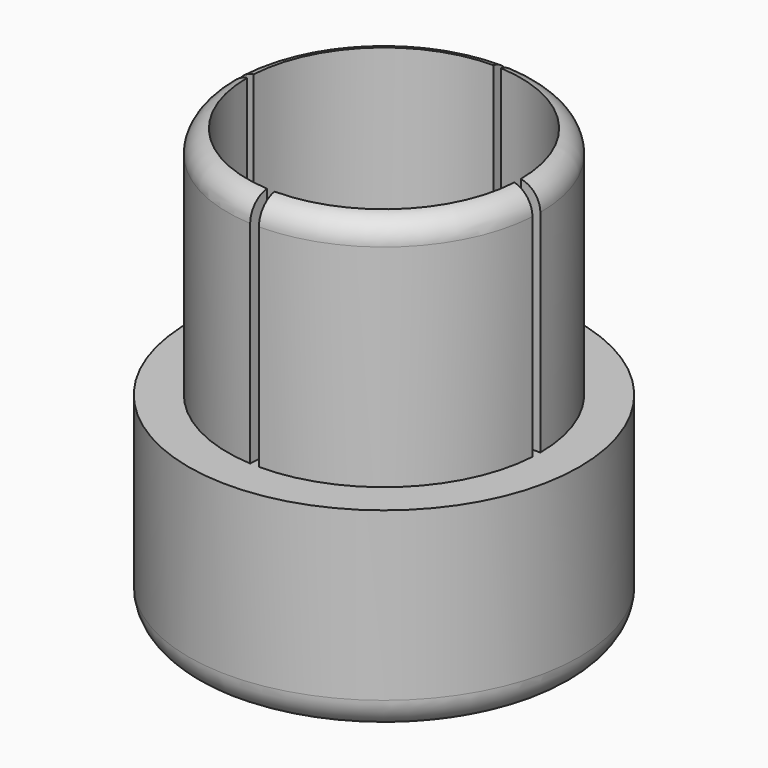
from build123d import *

# Parameters (mm, degrees)
F0_R        = 25
F0_R_2      = 20
F0_R_3      = 17.5
F1_DEPTH    = 25.4
F2_DEPTH    = 55.4
F4_DEPTH    = 30
F5_T2_ANGLE = 128.886649626
F5_T4_ANGLE = 129.1121145727
F5_T6_ANGLE = 128.886649626
F5_T8_ANGLE = 129.1121145727
F6_R        = 4


# Not quite as in the source:
# - a fillet or chamfer that OpenCascade refuses, or shapes differently, is made with other operations: its cross-section is extruded or revolved along the edge and cut away or added


with BuildPart() as f1:
    # F0 (on Top) → F1 (new body)
    with BuildSketch(Plane.XY):
        Circle(F0_R)
        Circle(F0_R_2, mode=Mode.SUBTRACT)
        Circle(F0_R_2)
        Circle(F0_R_3, mode=Mode.SUBTRACT)
    extrude(amount=F1_DEPTH)

    # F0 (on Top) → F2 (join)
    with BuildSketch(Plane.XY):
        Circle(F0_R_2)
        Circle(F0_R_3, mode=Mode.SUBTRACT)
    extrude(amount=F2_DEPTH)

    # F3 (on face) → F4 (cut)
    with BuildSketch(Plane.XY.offset(55.4)):
        with BuildLine():
            Line((0, 20), (0, 17.5))
            ThreePointArc((0, 17.5), (0.5, 17.4928556845), (0.9995917534, 17.4714285714))
            Line((0.9995917534, 17.4714285714), (1.1423905753, 19.9673469388))
            ThreePointArc((1.1423905753, 19.9673469388), (0.5714285714, 19.991835068), (0, 20))
        make_face()
        with BuildLine():
            Line((20, 0), (17.5, 0))
            ThreePointArc((17.5, 0), (17.4928556845, -0.5), (17.4714285714, -0.9995917534))
            Line((17.4714285714, -0.9995917534), (19.9626986738, -1.2209265568))
            ThreePointArc((19.9626986738, -1.2209265568), (19.9906724934, -0.6107481163), (20, 0))
        make_face()
        with BuildLine():
            ThreePointArc((-17.5, 0), (-17.4928556845, 0.5), (-17.4714285714, 0.9995917534))
            Line((-17.4714285714, 0.9995917534), (-19.9626986738, 1.2209265568))
            ThreePointArc((-19.9626986738, 1.2209265568), (-19.9906724934, 0.6107481163), (-20, 0))
            Line((-20, 0), (-17.5, 0))
        make_face()
        with BuildLine():
            ThreePointArc((0, -17.5), (-0.5, -17.4928556845), (-0.9995917534, -17.4714285714))
            Line((-0.9995917534, -17.4714285714), (-1.1423905753, -19.9673469388))
            ThreePointArc((-1.1423905753, -19.9673469388), (-0.5714285714, -19.991835068), (0, -20))
            Line((0, -20), (0, -17.5))
        make_face()
    extrude(amount=-F4_DEPTH, mode=Mode.SUBTRACT)

    # F5: fillet of radius 3 on 4 edges, made by hand

    # F5_s1 → F5_t2 (revolve, cut)
    with BuildSketch(Plane(origin=(0, 0, 0), x_dir=(0, 0, 1), z_dir=(0.9323663261, -0.3615149152, 0))):
        with BuildLine():
            ThreePointArc((52.4419601084, -20), (54.3784517816, -19.2912878475), (55.4, -17.5))
            Line((55.4, -17.5), (55.4, -20))
            Line((55.4, -20), (52.4419601084, -20))
        make_face()
    revolve(axis=Axis((0, 0, 55.4), (0, 0, 1)), revolution_arc=F5_T2_ANGLE, mode=Mode.SUBTRACT)

    # F5_s3 → F5_t4 (revolve, cut)
    with BuildSketch(Plane(origin=(0, 0, 0), x_dir=(0, 0, 1), z_dir=(0.3615155829, 0.9323660672, 0))):
        with BuildLine():
            ThreePointArc((52.4419601084, -20), (54.3784517816, -19.2912878475), (55.4, -17.5))
            Line((55.4, -17.5), (55.4, -20))
            Line((55.4, -20), (52.4419601084, -20))
        make_face()
    revolve(axis=Axis((0, 0, 55.4), (0, 0, 1)), revolution_arc=F5_T4_ANGLE, mode=Mode.SUBTRACT)

    # F5_s5 → F5_t6 (revolve, cut)
    with BuildSketch(Plane(origin=(0, 0, 0), x_dir=(0, 0, 1), z_dir=(-0.9323663261, 0.3615149152, 0))):
        with BuildLine():
            ThreePointArc((52.4419601084, -20), (54.3784517816, -19.2912878475), (55.4, -17.5))
            Line((55.4, -17.5), (55.4, -20))
            Line((55.4, -20), (52.4419601084, -20))
        make_face()
    revolve(axis=Axis((0, 0, 55.4), (0, 0, 1)), revolution_arc=F5_T6_ANGLE, mode=Mode.SUBTRACT)

    # F5_s7 → F5_t8 (revolve, cut)
    with BuildSketch(Plane(origin=(0, 0, 0), x_dir=(0, 0, 1), z_dir=(-0.3615155829, -0.9323660672, 0))):
        with BuildLine():
            ThreePointArc((52.4419601084, -20), (54.3784517816, -19.2912878475), (55.4, -17.5))
            Line((55.4, -17.5), (55.4, -20))
            Line((55.4, -20), (52.4419601084, -20))
        make_face()
    revolve(axis=Axis((0, 0, 55.4), (0, 0, 1)), revolution_arc=F5_T8_ANGLE, mode=Mode.SUBTRACT)

    # F6
    f6_edges = [f1.edges().sort_by_distance(p)[0] for p in [
        (-25, 0, 0),
    ]]
    fillet(f6_edges, radius=F6_R)


solid = f1.part
